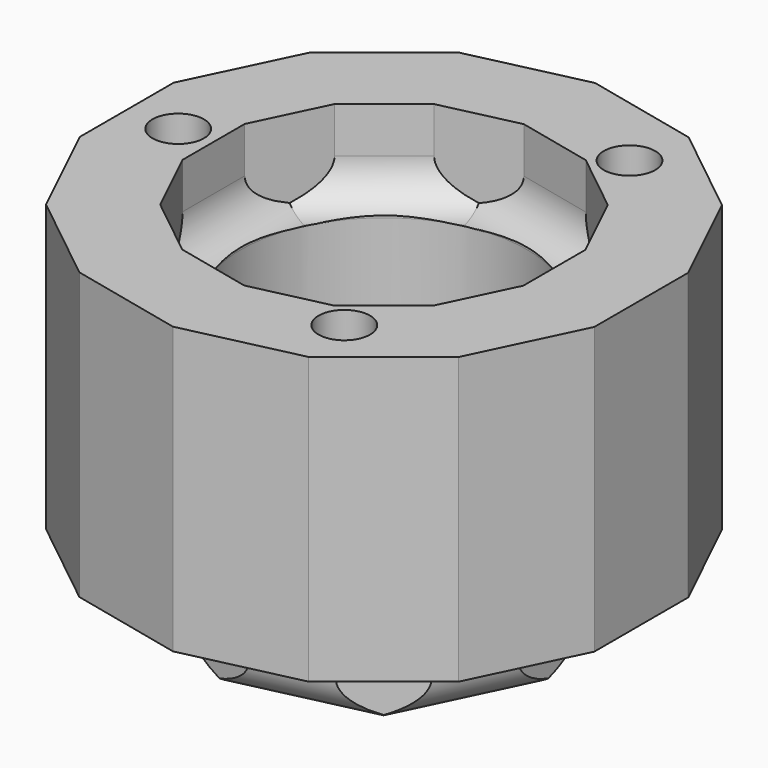
from build123d import *

# Parameters (mm, degrees)
F0_R         = 12.5
F1_DEPTH     = 12.5
F2_R         = 2.25
F3_DEPTH     = 25
F4_R         = 12.5
F5_DEPTH     = 7.5
F6_R         = 12.5
F7_DEPTH     = 7.5
F8_T4_DEPTH  = 24.3016555368
F8_S5_R      = 12.5
F8_T6_DEPTH  = 15
F8_T11_DEPTH = 24.3016555368
F8_S12_R     = 12.5
F8_T13_DEPTH = 14
F8_T17_DEPTH = 24.3016555368
F8_S18_R     = 12.5
F8_T19_DEPTH = 15
F8_T24_DEPTH = 24.3016555368
F8_S25_R     = 12.5
F8_T26_DEPTH = 15
F8_T30_DEPTH = 24.3016555368
F8_S31_R     = 12.5
F8_T32_DEPTH = 15
F8_T37_DEPTH = 24.3016555368
F8_S38_R     = 12.5
F8_T39_DEPTH = 15
F8_T44_DEPTH = 24.3016555368
F8_S45_R     = 12.5
F8_T46_DEPTH = 15
F9_T1_DEPTH  = 24.050587715
F9_T3_DEPTH  = 24.050587715
F9_T5_DEPTH  = 24.050587715
F9_T7_DEPTH  = 24.050587715
F9_T9_DEPTH  = 24.050587715
F9_T11_DEPTH = 24.050587715
F9_T13_DEPTH = 24.050587715


# Not quite as in the source:
# - a fillet or chamfer that OpenCascade refuses, or shapes differently, is made with other operations: its cross-section is extruded or revolved along the edge and cut away or added


with BuildPart() as f1:
    # F0 (on Top) → F1 (new body, symmetric)
    with BuildSketch(Plane.XY):
        Polygon((22.5, -5.1354781738), (22.5, 5.1354781738), (18.0435990556, 14.3892900865), (10.013442028, 20.7931266245), (0, 23.0786294236), (-10.013442028, 20.7931266245), (-18.0435990556, 14.3892900865), (-22.5, 5.1354781738), (-22.5, -5.1354781738), (-18.0435990556, -14.3892900865), (-10.013442028, -20.7931266245), (0, -23.0786294236), (10.013442028, -20.7931266245), (18.0435990556, -14.3892900865), align=None)
        Circle(F0_R, mode=Mode.SUBTRACT)
    extrude(amount=F1_DEPTH, both=True)

    # F2 (on face) → F3 (cut)
    with BuildSketch(Plane.XY.offset(12.5)):
        with Locations((9, 15.5884572681)):
            Circle(F2_R)
        with Locations((-18, 0)):
            Circle(F2_R)
        with Locations((9, -15.5884572681)):
            Circle(F2_R)
    extrude(amount=-F3_DEPTH, mode=Mode.SUBTRACT)

    # F4 (on face) → F5 (cut)
    with BuildSketch(Plane.XY.offset(12.5)):
        Polygon((14.9, -3.4008277684), (14.9, 3.4008277684), (11.9488722635, 9.5289076573), (6.6311238319, 13.7696705203), (0, 15.2831812628), (-6.6311238319, 13.7696705203), (-11.9488722635, 9.5289076573), (-14.9, 3.4008277684), (-14.9, -3.4008277684), (-11.9488722635, -9.5289076573), (-6.6311238319, -13.7696705203), (0, -15.2831812628), (6.6311238319, -13.7696705203), (11.9488722635, -9.5289076573), align=None)
        Circle(F4_R, mode=Mode.SUBTRACT)
    extrude(amount=-F5_DEPTH, mode=Mode.SUBTRACT)

    # F6 (on face) → F7 (join)
    with BuildSketch(Plane(origin=(0, 0, -12.5), x_dir=(1, 0, 0), z_dir=(0, 0, -1))):
        Polygon((14.35, -3.2752938575), (14.35, 3.2752938575), (11.5078065088, 9.1771694552), (6.3863508045, 13.2613940917), (0, 14.719036988), (-6.3863508045, 13.2613940917), (-11.5078065088, 9.1771694552), (-14.35, 3.2752938575), (-14.35, -3.2752938575), (-11.5078065088, -9.1771694552), (-6.3863508045, -13.2613940917), (0, -14.719036988), (6.3863508045, -13.2613940917), (11.5078065088, -9.1771694552), align=None)
        Circle(F6_R, mode=Mode.SUBTRACT)
    extrude(amount=F7_DEPTH)

    # F8: fillet of radius 3.5 on 7 edges, made by hand


with BuildPart() as f8_tool2:
    # F8_s3 → F8_t4 (new body)
    with BuildSketch(Plane(origin=(9.4998996874, 7.5759171977, 0), x_dir=(0, 0, 1), z_dir=(-0.7818314825, -0.6234898019, 0))):
        with BuildLine():
            ThreePointArc((5, 11.4), (6.0251262658, 13.8748737342), (8.5, 14.9))
            Line((8.5, 14.9), (5, 14.9))
            Line((5, 14.9), (5, 11.4))
        make_face()
    extrude(amount=F8_T4_DEPTH)

    # F8_s5 → F8_t6 (cut, symmetric)
    with BuildSketch(Plane.XY.offset(6.8)):
        Circle(F8_S5_R)
    extrude(amount=F8_T6_DEPTH, both=True, mode=Mode.SUBTRACT)

    split(bisect_by=Plane(origin=(-13.4244361317, 6.4648677129, 0), x_dir=(0, 0, 1), z_dir=(0.9009688679, -0.4338837391, 0)), keep=Keep.TOP)


with BuildPart() as f1_1:
    add(f1.part)

    # F8_t1: union F8_tool2
    add(f8_tool2.part)


with BuildPart() as f8_tool9:
    # F8_s10 → F8_t11 (new body)
    with BuildSketch(Plane.XZ.offset(-12.1508277684)):
        with BuildLine():
            ThreePointArc((-11.4, 5), (-13.8748737342, 6.0251262658), (-14.9, 8.5))
            Line((-14.9, 8.5), (-14.9, 5))
            Line((-14.9, 5), (-11.4, 5))
        make_face()
    extrude(amount=F8_T11_DEPTH)

    # F8_s12 → F8_t13 (cut, symmetric)
    with BuildSketch(Plane.XY.offset(6.8)):
        Circle(F8_S12_R)
    extrude(amount=F8_T13_DEPTH, both=True, mode=Mode.SUBTRACT)


with BuildPart() as f1_2:
    add(f1_1.part)

    # F8_t8: union F8_tool9
    add(f8_tool9.part)


with BuildPart() as f8_tool15:
    # F8_s16 → F8_t17 (new body)
    with BuildSketch(Plane(origin=(-9.4998996874, 7.5759171977, 0), x_dir=(0, 0, 1), z_dir=(0.7818314825, -0.6234898019, 0))):
        with BuildLine():
            ThreePointArc((5, 11.4), (6.0251262658, 13.8748737342), (8.5, 14.9))
            Line((8.5, 14.9), (5, 14.9))
            Line((5, 14.9), (5, 11.4))
        make_face()
    extrude(amount=F8_T17_DEPTH)

    # F8_s18 → F8_t19 (cut, symmetric)
    with BuildSketch(Plane.XY.offset(6.8)):
        Circle(F8_S18_R)
    extrude(amount=F8_T19_DEPTH, both=True, mode=Mode.SUBTRACT)

    split(bisect_by=Plane.YZ.offset(-14.9), keep=Keep.TOP)


with BuildPart() as f1_3:
    add(f1_2.part)

    # F8_t14: union F8_tool15
    add(f8_tool15.part)


with BuildPart() as f8_tool22:
    # F8_s23 → F8_t24 (new body)
    with BuildSketch(Plane(origin=(-11.8461811475, -2.7038135434, 0), x_dir=(0, 0, 1), z_dir=(0.9749279122, 0.222520934, 0))):
        with BuildLine():
            ThreePointArc((8.5, 14.9), (6.0251262658, 13.8748737342), (5, 11.4))
            Line((5, 11.4), (5, 14.9))
            Line((5, 14.9), (8.5, 14.9))
        make_face()
    extrude(amount=F8_T24_DEPTH)

    # F8_s25 → F8_t26 (cut, symmetric)
    with BuildSketch(Plane.XY.offset(6.8)):
        Circle(F8_S25_R)
    extrude(amount=F8_T26_DEPTH, both=True, mode=Mode.SUBTRACT)


with BuildPart() as f1_4:
    add(f1_3.part)

    # F8_t21: union F8_tool22
    add(f8_tool22.part)


with BuildPart() as f8_tool28:
    # F8_s29 → F8_t30 (new body)
    with BuildSketch(Plane(origin=(-5.2720465855, -10.9475175386, 0), x_dir=(0, 0, 1), z_dir=(0.4338837391, 0.9009688679, 0))):
        with BuildLine():
            ThreePointArc((5, 11.4), (6.0251262658, 13.8748737342), (8.5, 14.9))
            Line((8.5, 14.9), (5, 14.9))
            Line((5, 14.9), (5, 11.4))
        make_face()
    extrude(amount=F8_T30_DEPTH)

    # F8_s31 → F8_t32 (cut, symmetric)
    with BuildSketch(Plane.XY.offset(6.8)):
        Circle(F8_S31_R)
    extrude(amount=F8_T32_DEPTH, both=True, mode=Mode.SUBTRACT)

    split(bisect_by=Plane(origin=(9.2899980477, -11.6492890888, 0), x_dir=(0, 0, 1), z_dir=(-0.6234898019, 0.7818314825, 0)), keep=Keep.TOP)


with BuildPart() as f1_5:
    add(f1_4.part)

    # F8_t27: union F8_tool28
    add(f8_tool28.part)


with BuildPart() as f8_tool35:
    # F8_s36 → F8_t37 (new body)
    with BuildSketch(Plane(origin=(5.2720465855, -10.9475175386, 0), x_dir=(0, 0, 1), z_dir=(-0.4338837391, 0.9009688679, 0))):
        with BuildLine():
            ThreePointArc((5, 11.4), (6.0251262658, 13.8748737342), (8.5, 14.9))
            Line((8.5, 14.9), (5, 14.9))
            Line((5, 14.9), (5, 11.4))
        make_face()
    extrude(amount=F8_T37_DEPTH)

    # F8_s38 → F8_t39 (cut, symmetric)
    with BuildSketch(Plane.XY.offset(6.8)):
        Circle(F8_S38_R)
    extrude(amount=F8_T39_DEPTH, both=True, mode=Mode.SUBTRACT)

    split(bisect_by=Plane(origin=(9.2899980477, 11.6492890888, 0), x_dir=(0, 0, 1), z_dir=(-0.6234898019, -0.7818314825, 0)), keep=Keep.TOP)


with BuildPart() as f1_6:
    add(f1_5.part)

    # F8_t34: union F8_tool35
    add(f8_tool35.part)


with BuildPart() as f8_tool42:
    # F8_s43 → F8_t44 (new body)
    with BuildSketch(Plane(origin=(11.8461811475, -2.7038135434, 0), x_dir=(0, 0, 1), z_dir=(-0.9749279122, 0.222520934, 0))):
        with BuildLine():
            ThreePointArc((5, 11.4), (6.0251262658, 13.8748737342), (8.5, 14.9))
            Line((8.5, 14.9), (5, 14.9))
            Line((5, 14.9), (5, 11.4))
        make_face()
    extrude(amount=F8_T44_DEPTH)

    # F8_s45 → F8_t46 (cut, symmetric)
    with BuildSketch(Plane.XY.offset(6.8)):
        Circle(F8_S45_R)
    extrude(amount=F8_T46_DEPTH, both=True, mode=Mode.SUBTRACT)


with BuildPart() as f1_7:
    add(f1_6.part)

    # F8_t41: union F8_tool42
    add(f8_tool42.part)

    # F9: fillet of radius 3.5 on 7 edges, made by hand

    # F9_s2 → F9_t1 (cut)
    with BuildSketch(Plane(origin=(-5.2175794629, 10.834415393, 0), x_dir=(0, 0, 1), z_dir=(0.4338837391, -0.9009688679, 0))):
        with BuildLine():
            ThreePointArc((-16.5, -14.35), (-18.9748737342, -13.3248737342), (-20, -10.85))
            Line((-20, -10.85), (-20, -14.35))
            Line((-20, -14.35), (-16.5, -14.35))
        make_face()
    extrude(amount=F9_T1_DEPTH, mode=Mode.SUBTRACT)

    # F9_s4 → F9_t3 (cut)
    with BuildSketch(Plane(origin=(-11.7237946339, 2.6758796203, 0), x_dir=(0, 0, 1), z_dir=(0.9749279122, -0.222520934, 0))):
        with BuildLine():
            ThreePointArc((-16.5, -14.35), (-18.9748737342, -13.3248737342), (-20, -10.85))
            Line((-20, -10.85), (-20, -14.35))
            Line((-20, -14.35), (-16.5, -14.35))
        make_face()
    extrude(amount=F9_T3_DEPTH, mode=Mode.SUBTRACT)

    # F9_s6 → F9_t5 (cut)
    with BuildSketch(Plane(origin=(-9.4017533237, -7.4976480845, 0), x_dir=(0, 0, 1), z_dir=(0.7818314825, 0.6234898019, 0))):
        with BuildLine():
            ThreePointArc((-16.5, -14.35), (-18.9748737342, -13.3248737342), (-20, -10.85))
            Line((-20, -10.85), (-20, -14.35))
            Line((-20, -14.35), (-16.5, -14.35))
        make_face()
    extrude(amount=F9_T5_DEPTH, mode=Mode.SUBTRACT)

    # F9_s8 → F9_t7 (cut)
    with BuildSketch(Plane.XZ.offset(-12.0252938575)):
        with BuildLine():
            ThreePointArc((-14.35, -16.5), (-13.3248737342, -18.9748737342), (-10.85, -20))
            Line((-10.85, -20), (-14.35, -20))
            Line((-14.35, -20), (-14.35, -16.5))
        make_face()
    extrude(amount=F9_T7_DEPTH, mode=Mode.SUBTRACT)

    # F9_s10 → F9_t9 (cut)
    with BuildSketch(Plane(origin=(9.4017533237, -7.4976480845, 0), x_dir=(0, 0, 1), z_dir=(-0.7818314825, 0.6234898019, 0))):
        with BuildLine():
            ThreePointArc((-16.5, -14.35), (-18.9748737342, -13.3248737342), (-20, -10.85))
            Line((-20, -10.85), (-20, -14.35))
            Line((-20, -14.35), (-16.5, -14.35))
        make_face()
    extrude(amount=F9_T9_DEPTH, mode=Mode.SUBTRACT)

    # F9_s12 → F9_t11 (cut)
    with BuildSketch(Plane(origin=(11.7237946339, 2.6758796203, 0), x_dir=(0, 0, 1), z_dir=(-0.9749279122, -0.222520934, 0))):
        with BuildLine():
            ThreePointArc((-16.5, -14.35), (-18.9748737342, -13.3248737342), (-20, -10.85))
            Line((-20, -10.85), (-20, -14.35))
            Line((-20, -14.35), (-16.5, -14.35))
        make_face()
    extrude(amount=F9_T11_DEPTH, mode=Mode.SUBTRACT)

    # F9_s14 → F9_t13 (cut)
    with BuildSketch(Plane(origin=(5.2175794629, 10.834415393, 0), x_dir=(0, 0, 1), z_dir=(-0.4338837391, -0.9009688679, 0))):
        with BuildLine():
            ThreePointArc((-16.5, -14.35), (-18.9748737342, -13.3248737342), (-20, -10.85))
            Line((-20, -10.85), (-20, -14.35))
            Line((-20, -14.35), (-16.5, -14.35))
        make_face()
    extrude(amount=F9_T13_DEPTH, mode=Mode.SUBTRACT)


solid = f1_7.part
